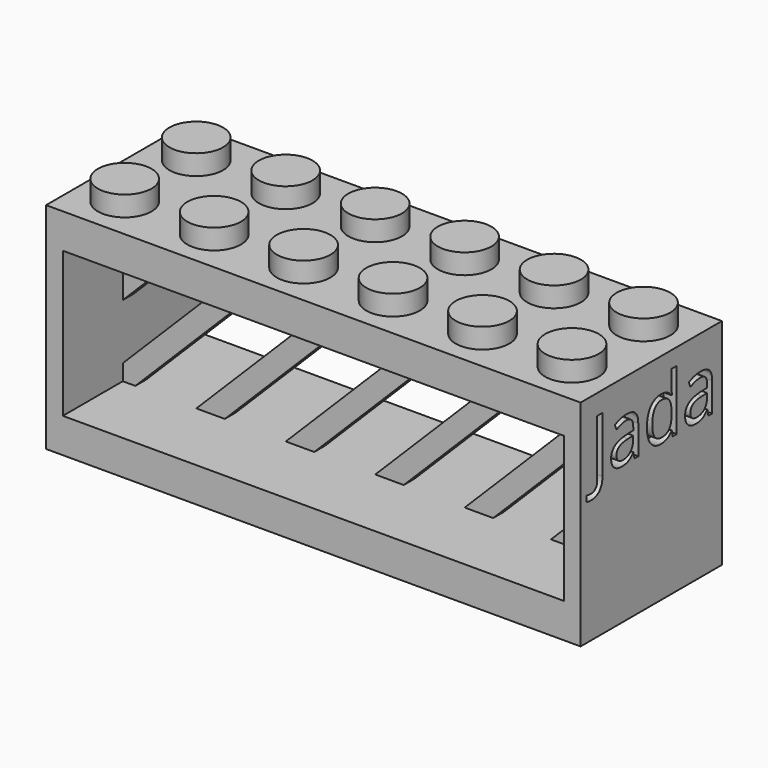
from build123d import *

# Parameters (mm, degrees)
F0_W          = 47.8
F0_H          = 15.8
F1_DEPTH      = 19.2
F2_W          = 45.4
F2_H          = 13.4
F3_DEPTH      = 1.9
F4_W          = 44.8
F4_H          = 13
F5_DEPTH      = 15.8
F7_DEPTH      = 1.2
F8_R          = 2.4
F9_DEPTH      = 1.8
F10_R         = 3.255
F10_R_2       = 2.4
F11_DEPTH     = 1.9
F12_W         = 0.6
F12_H         = 0.3
F14_DEPTH     = 1.9
F15_W         = 0.3
F15_H         = 0.6
F16_DEPTH     = 1.9
F17_TEXT_SIZE = 7.0690927613
F18_DEPTH     = 1.2


# Not quite as in the source:
# - Text() gives the source's letters only with a copy of the font that has no kerning and outlines rounded to 1/6400 em; it was checked with that copy


with BuildPart() as f1:
    # F0 (on Top) → F1 (new body)
    with BuildSketch(Plane.XY):
        Rectangle(F0_W, F0_H)
    extrude(amount=F1_DEPTH)

    # F2 (on face) → F3 (cut)
    with BuildSketch(Plane(origin=(0, 0, 0), x_dir=(1, 0, 0), z_dir=(0, 0, -1))):
        Rectangle(F2_W, F2_H)
    extrude(amount=-F3_DEPTH, mode=Mode.SUBTRACT)

    # F4 (on face) → F5 (cut)
    with BuildSketch(Plane.XZ.offset(7.9)):
        with Locations((0, 9.6)):
            Rectangle(F4_W, F4_H)
    extrude(amount=-F5_DEPTH, mode=Mode.SUBTRACT)

    # F6 (on Front) → F7 (join)
    with BuildSketch(Plane.XZ):
        Polygon((-15.3155378891, 19.1213413087), (-23.7968791978, 10.64), (-23.7063318188, 8.1849629668), (-13.0763725055, 18.8149222801), align=None)
        Polygon((15.5137548597, 2.7193392719), (18.0593392719, 2.7193392719), (23.5820666091, 8.2420666091), (23.813447088, 11.0190315003), align=None)
        Polygon((-6.7624578107, 17.6131145708), (-9.1264915249, 17.794665269), (-22.8033869295, 4.1177698644), (-23.0306496611, 2.6177149266), (-21.757857455, 2.6177149266), align=None)
        Polygon((1.2375421893, 17.6131145708), (-1.1264915249, 17.794665269), (-14.8033869295, 4.1177698644), (-16.3034418672, 2.6177149266), (-13.757857455, 2.6177149266), align=None)
        Polygon((9.2375421893, 17.6131145708), (6.8735084751, 17.794665269), (-6.8033869295, 4.1177698644), (-8.3034418672, 2.6177149266), (-5.757857455, 2.6177149266), align=None)
        Polygon((17.2375421893, 17.6131145708), (14.8735084751, 17.794665269), (1.1966130705, 4.1177698644), (-0.3034418672, 2.6177149266), (2.242142545, 2.6177149266), align=None)
        Polygon((23.2509010555, 15.6264734371), (22.8735084751, 17.794665269), (9.1966130705, 4.1177698644), (7.6965581328, 2.6177149266), (10.242142545, 2.6177149266), align=None)
    extrude(amount=F7_DEPTH)

    # F8 (on face) → F9 (join)
    with BuildSketch(Plane.XY.offset(19.2)):
        with Locations((-19.95, 3.95)):
            Circle(F8_R)
        with Locations((-19.95, -4.05)):
            Circle(F8_R)
        with Locations((-11.95, 3.95)):
            Circle(F8_R)
        with Locations((-11.95, -4.05)):
            Circle(F8_R)
        with Locations((-3.95, 3.95)):
            Circle(F8_R)
        with Locations((-3.95, -4.05)):
            Circle(F8_R)
        with Locations((4.05, 3.95)):
            Circle(F8_R)
        with Locations((4.05, -4.05)):
            Circle(F8_R)
        with Locations((12.05, 3.95)):
            Circle(F8_R)
        with Locations((12.05, -4.05)):
            Circle(F8_R)
        with Locations((20.05, 3.95)):
            Circle(F8_R)
        with Locations((20.05, -4.05)):
            Circle(F8_R)
    extrude(amount=F9_DEPTH)

    # F10 (on face) → F11 (join, through all)
    with BuildSketch(Plane(origin=(0, 0, 1.9), x_dir=(1, 0, 0), z_dir=(0, 0, -1))):
        with Locations((16.05, -0.05)):
            Circle(F10_R)
        with Locations((16.05, -0.05)):
            Circle(F10_R_2, mode=Mode.SUBTRACT)
        with Locations((8.05, -0.05)):
            Circle(F10_R)
        with Locations((8.05, -0.05)):
            Circle(F10_R_2, mode=Mode.SUBTRACT)
        with Locations((0.05, -0.05)):
            Circle(F10_R)
        Circle(F10_R_2, mode=Mode.SUBTRACT)
        with Locations((-7.95, 0)):
            Circle(F10_R)
        with Locations((-7.95, 0)):
            Circle(F10_R_2, mode=Mode.SUBTRACT)
        with Locations((-15.95, -0.05)):
            Circle(F10_R)
        with Locations((-15.95, -0.05)):
            Circle(F10_R_2, mode=Mode.SUBTRACT)
    extrude(amount=F11_DEPTH)

    # F12 (on face) → F14 (join, through all)
    with BuildSketch(Plane(origin=(0, 0, 1.9), x_dir=(1, 0, 0), z_dir=(0, 0, -1))):
        with Locations((-19.95, 6.55)):
            Rectangle(F12_W, F12_H)
        with Locations((-19.95, -6.55)):
            Rectangle(F12_W, F12_H)
        with Locations((-11.95, 6.55)):
            Rectangle(F12_W, F12_H)
        with Locations((-11.95, -6.55)):
            Rectangle(F12_W, F12_H)
        with Locations((-3.95, 6.55)):
            Rectangle(F12_W, F12_H)
        with Locations((-3.95, -6.55)):
            Rectangle(F12_W, F12_H)
        with Locations((4.05, 6.55)):
            Rectangle(F12_W, F12_H)
        with Locations((4.05, -6.55)):
            Rectangle(F12_W, F12_H)
        with Locations((12.05, 6.55)):
            Rectangle(F12_W, F12_H)
        with Locations((12.05, -6.55)):
            Rectangle(F12_W, F12_H)
        with Locations((20.05, 6.55)):
            Rectangle(F12_W, F12_H)
        with Locations((20.05, -6.55)):
            Rectangle(F12_W, F12_H)
    extrude(amount=F14_DEPTH)

    # F15 (on face) → F16 (join, through all)
    with BuildSketch(Plane(origin=(0, 0, 1.9), x_dir=(1, 0, 0), z_dir=(0, 0, -1))):
        with Locations((-22.55, 3.95)):
            Rectangle(F15_W, F15_H)
        with Locations((-22.55, -4.05)):
            Rectangle(F15_W, F15_H)
        with Locations((22.55, 3.95)):
            Rectangle(F15_W, F15_H)
        with Locations((22.55, -4.05)):
            Rectangle(F15_W, F15_H)
    extrude(amount=F16_DEPTH)

    # F17 (on face) → F18 (cut)
    with BuildSketch(Plane.YZ.offset(23.9)):
        with Locations((-6.6978680552, 12.3530011624)):
            Text('Jada', F17_TEXT_SIZE, font='Open Sans', text_align=(TextAlign.LEFT, TextAlign.BOTTOM))
    extrude(amount=-F18_DEPTH, mode=Mode.SUBTRACT)


solid = f1.part
